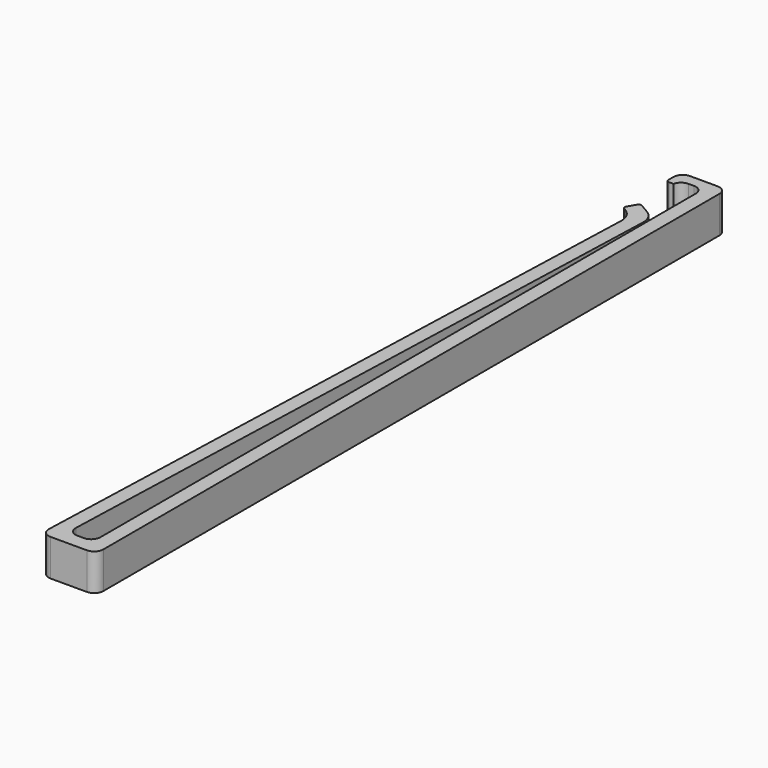
from build123d import *

# Parameters (mm, degrees)
F1_DEPTH     = 4
F2_R         = 2
F3_T1_DEPTH  = 4
F3_T3_DEPTH  = 4
F3_T5_DEPTH  = 4
F3_T7_DEPTH  = 4
F3_T9_DEPTH  = 9.1726954634
F3_T11_DEPTH = 9
F3_T13_DEPTH = 9
F3_T15_DEPTH = 9
F4_R         = 0.3
F5_TEXT_SIZE = 3.4722222222
F6_DEPTH     = 0.5


# Not quite as in the source:
# - a fillet or chamfer that OpenCascade refuses, or shapes differently, is made with other operations: its cross-section is extruded or revolved along the edge and cut away or added
# - Text() gives the source's letters only with a copy of the font that has no kerning and outlines rounded to 1/6400 em; it was checked with that copy


with BuildPart() as f1:
    # F0 (on Top) → F1 (new body)
    with BuildSketch(Plane.XY):
        Polygon((2.6183253452, 77.0945269398), (0, 0), (1.6009224969, 0), (6, 0), (6, 86), (1, 86), (1, 84), (1.8, 84), (1.8, 84.8), (4.4, 84.8), (4.4, 1.6), (1.6552625483, 1.6), (4.25, 78), (1.923438968, 79.3432406381), (1.123438968, 77.9575999921), align=None)
    extrude(amount=F1_DEPTH)

    # F2
    f2_edges = [f1.edges().sort_by_distance(p)[0] for p in [
        (4.25, 78, 2),
        (2.618325, 77.094527, 2),
    ]]
    fillet(f2_edges, radius=F2_R)

    # F3: fillet of radius 1 on 8 edges, made by hand

    # F3_s2 → F3_t1 (join)
    with BuildSketch(Plane.XY):
        with BuildLine():
            ThreePointArc((1.6903778693, 2.6339429619), (1.9707943524, 1.9049974683), (2.6898016409, 1.6))
            Line((2.6898016409, 1.6), (1.6552625483, 1.6))
            Line((1.6552625483, 1.6), (1.6903778693, 2.6339429619))
        make_face()
    extrude(amount=F3_T1_DEPTH)

    # F3_s4 → F3_t3 (join)
    with BuildSketch(Plane.XY):
        with BuildLine():
            ThreePointArc((3.4, 1.6), (4.1071067812, 1.8928932188), (4.4, 2.6))
            Line((4.4, 2.6), (4.4, 1.6))
            Line((4.4, 1.6), (3.4, 1.6))
        make_face()
    extrude(amount=F3_T3_DEPTH)

    # F3_s6 → F3_t5 (join)
    with BuildSketch(Plane.XY):
        with BuildLine():
            ThreePointArc((3.4, 84.8), (4.1071067812, 84.5071067812), (4.4, 83.8))
            Line((4.4, 83.8), (4.4, 84.8))
            Line((4.4, 84.8), (3.4, 84.8))
        make_face()
    extrude(amount=F3_T5_DEPTH)

    # F3_s8 → F3_t7 (join)
    with BuildSketch(Plane.XY):
        with BuildLine():
            ThreePointArc((1.8, 84), (2.1473403651, 84.5745966692), (2.7797958971, 84.8))
            Line((2.7797958971, 84.8), (1.8, 84.8))
            Line((1.8, 84.8), (1.8, 84))
        make_face()
    extrude(amount=F3_T7_DEPTH)

    # F3_s10 → F3_t9 (cut)
    with BuildSketch(Plane.XY.offset(-2.5863477317)):
        with BuildLine():
            ThreePointArc((0.035115321, 1.0339429619), (0.3155318041, 0.3049974683), (1.0345390927, 0))
            Line((1.0345390927, 0), (0, 0))
            Line((0, 0), (0.035115321, 1.0339429619))
        make_face()
    extrude(amount=F3_T9_DEPTH, mode=Mode.SUBTRACT)

    # F3_s12 → F3_t11 (cut)
    with BuildSketch(Plane.XY.offset(-2.5)):
        with BuildLine():
            ThreePointArc((6, 1), (5.7071067812, 0.2928932188), (5, 0))
            Line((5, 0), (6, 0))
            Line((6, 0), (6, 1))
        make_face()
    extrude(amount=F3_T11_DEPTH, mode=Mode.SUBTRACT)

    # F3_s14 → F3_t13 (cut)
    with BuildSketch(Plane.XY.offset(-2.5)):
        with BuildLine():
            ThreePointArc((5, 86), (5.7071067812, 85.7071067812), (6, 85))
            Line((6, 85), (6, 86))
            Line((6, 86), (5, 86))
        make_face()
    extrude(amount=F3_T13_DEPTH, mode=Mode.SUBTRACT)

    # F3_s16 → F3_t15 (cut)
    with BuildSketch(Plane.XY.offset(-2.5)):
        with BuildLine():
            ThreePointArc((1, 85), (1.2928932188, 85.7071067812), (2, 86))
            Line((2, 86), (1, 86))
            Line((1, 86), (1, 85))
        make_face()
    extrude(amount=F3_T15_DEPTH, mode=Mode.SUBTRACT)

    # F4
    f4_edges = [f1.edges().sort_by_distance(p)[0] for p in [
        (1.923439, 79.343241, 2),
        (1.123439, 77.9576, 2),
        (1, 84, 2),
    ]]
    fillet(f4_edges, radius=F4_R)

    # F5 (on face) → F6 (cut)
    with BuildSketch(Plane(origin=(0, 0, 0), x_dir=(-0.0339429619, -0.9994237716, 0), z_dir=(-0.9994237716, 0.0339429619, 0))):
        with Locations((-53.6735026042, 0.9)):
            Text('MoneyPocket', F5_TEXT_SIZE, font='Open Sans', font_style=FontStyle.BOLD, text_align=(TextAlign.LEFT, TextAlign.BOTTOM))
    extrude(amount=-F6_DEPTH, mode=Mode.SUBTRACT)


solid = f1.part
